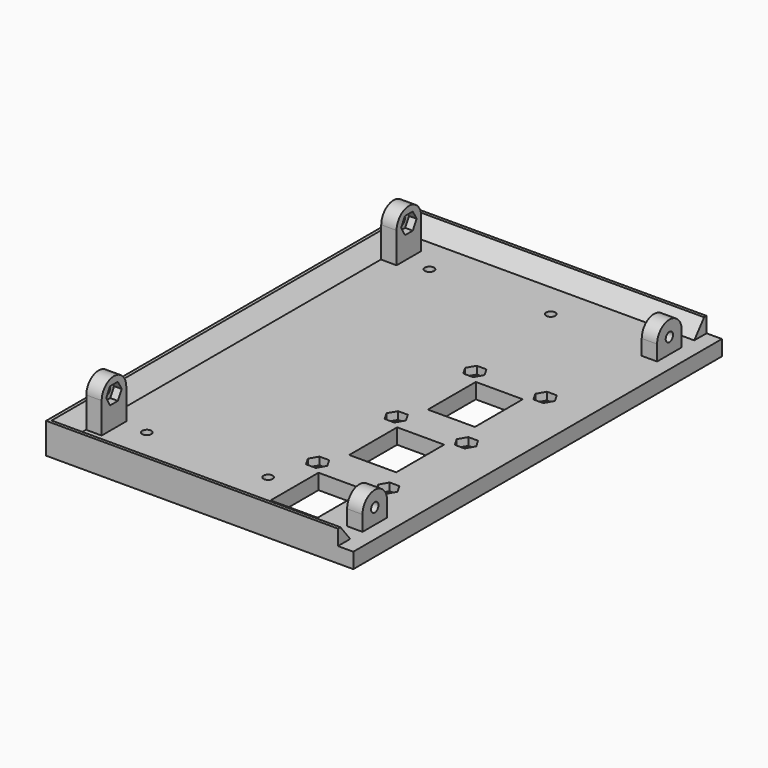
from build123d import *

# Parameters (mm, degrees)
F0_W            = 100
F0_H            = 150
F1_DEPTH        = 5
F5_DEPTH        = 150
F6_DEPTH        = 100
F7_W            = 5
F7_H            = 5
F8_DEPTH        = 160
F10_R           = 1.5
F11_DEPTH       = 25
F12_R           = 2.75
F13_DEPTH       = 2
F14_W           = 5
F14_H           = 10
F15_DEPTH       = 20
F16_R           = 1.5
F17_DEPTH       = 10
F18_R           = 1.5
F19_DEPTH       = 25
F21_DEPTH       = 2.5
F23_DEPTH       = 2.5
F25_DEPTH       = 2.5
F9_R            = 1.7
F9_W            = 15.3
F9_H            = 19.5
F26_DEPTH       = 25
F27_TEXT_SIZE   = 20.8333333333
F27_TEXT_SIZE_2 = 9.7222222222
F28_DEPTH       = 0.5


# Not quite as in the source:
# - Text() gives the source's letters only with a copy of the font that has no kerning and outlines rounded to 1/6400 em; it was checked with that copy


with BuildPart() as f1:
    # F0 (on Top) → F1 (new body)
    with BuildSketch(Plane.XY):
        Rectangle(F0_W, F0_H)
    extrude(amount=F1_DEPTH)

    # F3 (on face) → F5 (join)
    with BuildSketch(Plane.XZ.offset(75)):
        Polygon((-50, 10), (-50, 5), (-45, 5), (-49, 10), align=None)
    extrude(amount=-F5_DEPTH)

    # F4 (on face) → F6 (join)
    with BuildSketch(Plane.YZ.offset(50)):
        Polygon((-75, 10), (-75, 5), (-70, 5), (-74, 10), align=None)
        Polygon((75, 5), (75, 10), (74, 10), (70, 5), align=None)
    extrude(amount=-F6_DEPTH)

    # F7 (on face) → F8 (cut)
    with BuildSketch(Plane.XZ.offset(75)):
        with Locations((47.5, 7.5)):
            Rectangle(F7_W, F7_H)
    extrude(amount=-F8_DEPTH, mode=Mode.SUBTRACT)

    # F10 (on face) → F11 (cut)
    with BuildSketch(Plane(origin=(0, 0, 0), x_dir=(1, 0, 0), z_dir=(0, 0, -1))):
        with Locations((7.5, 56.5)):
            Circle(F10_R)
        with Locations((-32, -58.5)):
            Circle(F10_R)
        with Locations((7.5, -58.5)):
            Circle(F10_R)
        with Locations((-32, 56.5)):
            Circle(F10_R)
    extrude(amount=-F11_DEPTH, mode=Mode.SUBTRACT)

    # F12 (on face) → F13 (cut)
    with BuildSketch(Plane(origin=(0, 0, 0), x_dir=(1, 0, 0), z_dir=(0, 0, -1))):
        with Locations((-32, 56.5)):
            Circle(F12_R)
        with Locations((7.5, 56.5)):
            Circle(F12_R)
        with Locations((-32, -58.5)):
            Circle(F12_R)
        with Locations((7.5, -58.5)):
            Circle(F12_R)
    extrude(amount=-F13_DEPTH, mode=Mode.SUBTRACT)

    # F14 (on face) → F15 (join)
    with BuildSketch(Plane.XY.offset(5)):
        with Locations((-42.4, 60)):
            Rectangle(F14_W, F14_H)
        with Locations((42.4, 60)):
            Rectangle(F14_W, F14_H)
        with Locations((-42.4, -60)):
            Rectangle(F14_W, F14_H)
        with Locations((42.5, -60)):
            Rectangle(F14_W, F14_H)
    extrude(amount=F15_DEPTH)

    # F16 (on face) → F17 (cut)
    with BuildSketch(Plane.YZ.offset(45)):
        with Locations((-60, 10)):
            Circle(F16_R)
        with BuildLine():
            Line((-65, 25), (-65, 10))
            ThreePointArc((-65, 10), (-60, 15), (-55, 10))
            Line((-55, 10), (-55, 25))
            Line((-55, 25), (-65, 25))
        make_face()
        with Locations((60, 10)):
            Circle(F16_R)
        with BuildLine():
            Line((65, 25), (55, 25))
            Line((55, 25), (55, 10))
            ThreePointArc((55, 10), (60, 15), (65, 10))
            Line((65, 10), (65, 25))
        make_face()
    extrude(amount=-F17_DEPTH, mode=Mode.SUBTRACT)

    # F18 (on face) → F19 (cut)
    with BuildSketch(Plane.YZ.offset(-39.9)):
        with Locations((-60, 15)):
            Circle(F18_R)
        with BuildLine():
            ThreePointArc((-65, 15), (-60, 20), (-55, 15))
            Line((-55, 15), (-55, 25))
            Line((-55, 25), (-65, 25))
            Line((-65, 25), (-65, 15))
        make_face()
        with BuildLine():
            Line((55, 25), (55, 15))
            ThreePointArc((55, 15), (60, 20), (65, 15))
            Line((65, 15), (65, 25))
            Line((65, 25), (55, 25))
        make_face()
        with Locations((60, 15)):
            Circle(F18_R)
    extrude(amount=-F19_DEPTH, mode=Mode.SUBTRACT)

    # F20 (on face) → F21 (cut)
    with BuildSketch(Plane(origin=(40, 0, 0), x_dir=(0, -1, 0), z_dir=(-1, 0, 0))):
        Polygon((61.5877132403, 12.75), (58.4122867597, 12.75), (56.8245735195, 10), (58.4122867597, 7.25), (61.5877132403, 7.25), (63.1754264805, 10), align=None)
        Polygon((-58.4122867597, 7.25), (-56.8245735195, 10), (-58.4122867597, 12.75), (-61.5877132403, 12.75), (-63.1754264805, 10), (-61.5877132403, 7.25), align=None)
    extrude(amount=-F21_DEPTH, mode=Mode.SUBTRACT)

    # F22 (on face) → F23 (cut)
    with BuildSketch(Plane.YZ.offset(-39.9)):
        Polygon((-58.4122867597, 17.75), (-61.5877132403, 17.75), (-63.1754264805, 15), (-61.5877132403, 12.25), (-58.4122867597, 12.25), (-56.8245735195, 15), align=None)
        Polygon((61.5877132403, 12.25), (63.1754264805, 15), (61.5877132403, 17.75), (58.4122867597, 17.75), (56.8245735195, 15), (58.4122867597, 12.25), align=None)
    extrude(amount=-F23_DEPTH, mode=Mode.SUBTRACT)

    # F24 (on face) → F25 (cut)
    with BuildSketch(Plane.XY.offset(5)):
        Polygon((13.7277132403, 24.55), (10.5522867597, 24.55), (8.9645735195, 21.8), (10.5522867597, 19.05), (13.7277132403, 19.05), (15.3154264805, 21.8), align=None)
        Polygon((15.3154264805, -10.2), (13.7277132403, -7.45), (10.5522867597, -7.45), (8.9645735195, -10.2), (10.5522867597, -12.95), (13.7277132403, -12.95), align=None)
        Polygon((15.3154264805, -42.2), (13.7277132403, -39.45), (10.5522867597, -39.45), (8.9645735195, -42.2), (10.5522867597, -44.95), (13.7277132403, -44.95), align=None)
        Polygon((38.1754264805, 21.8), (36.5877132403, 24.55), (33.4122867597, 24.55), (31.8245735195, 21.8), (33.4122867597, 19.05), (36.5877132403, 19.05), align=None)
        Polygon((38.1754264805, -10.2), (36.5877132403, -7.45), (33.4122867597, -7.45), (31.8245735195, -10.2), (33.4122867597, -12.95), (36.5877132403, -12.95), align=None)
        Polygon((38.1754264805, -42.2), (36.5877132403, -39.45), (33.4122867597, -39.45), (31.8245735195, -42.2), (33.4122867597, -44.95), (36.5877132403, -44.95), align=None)
    extrude(amount=-F25_DEPTH, mode=Mode.SUBTRACT)

    # F9 (on face) → F26 (cut)
    with BuildSketch(Plane.XY.offset(5)):
        with Locations((35, 21.8)):
            Circle(F9_R)
        with Locations((12.14, 21.8)):
            Circle(F9_R)
        with Locations((23.57, 7.7)):
            Rectangle(F9_W, F9_H)
        with Locations((35, -10.2)):
            Circle(F9_R)
        with Locations((12.14, -10.2)):
            Circle(F9_R)
        with Locations((23.57, -24.3)):
            Rectangle(F9_W, F9_H)
        with Locations((35, -42.2)):
            Circle(F9_R)
        with Locations((12.14, -42.2)):
            Circle(F9_R)
        with Locations((23.57, -56.3)):
            Rectangle(F9_W, F9_H)
    extrude(amount=-F26_DEPTH, mode=Mode.SUBTRACT)

    # F27 (on face) → F28 (cut)
    with BuildSketch(Plane(origin=(0, 0, 0), x_dir=(1, 0, 0), z_dir=(0, 0, -1))):
        with Locations(Location((5.92, -0.2), (0, 0, 180))):
            Text('R', F27_TEXT_SIZE, font='Open Sans', text_align=(TextAlign.LEFT, TextAlign.BOTTOM))
        with Locations(Location((5.92, 31.8), (0, 0, 180))):
            Text('S', F27_TEXT_SIZE, font='Open Sans', text_align=(TextAlign.LEFT, TextAlign.BOTTOM))
        with Locations(Location((5.92, 63.8), (0, 0, 180))):
            Text('T', F27_TEXT_SIZE, font='Open Sans', text_align=(TextAlign.LEFT, TextAlign.BOTTOM))
        with Locations(Location((30.8595, -27.45), (0, 0, 180))):
            Text('F N', F27_TEXT_SIZE_2, font='Open Sans', text_align=(TextAlign.LEFT, TextAlign.BOTTOM))
    extrude(amount=-F28_DEPTH, mode=Mode.SUBTRACT)


solid = f1.part
